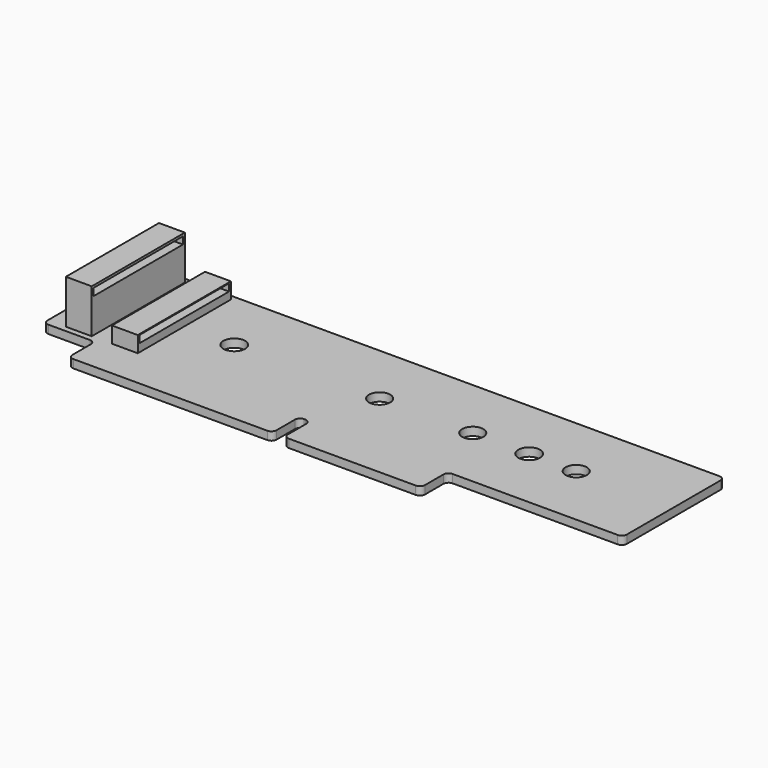
from build123d import *

# Parameters (mm, degrees)
F4_W         = 39.45
F4_H         = 6.43
F4_W_2       = 26.5
F4_R         = 2.105
F4_R_2       = 2.05
F5_DEPTH     = 1.6
F7_DEPTH     = 3.1
F6_W         = 5
F6_H         = 22.5
F8_DEPTH     = 8.5
F9_R         = 1
F10_W        = 21.6
F10_H        = 1.4
F11_DEPTH    = 3.1
F12_T1_DEPTH = 21.6
F13_W        = 21.6
F13_H        = 1.4
F14_DEPTH    = 3.1
F15_T1_DEPTH = 21.6


# Not quite as in the source:
# - a fillet or chamfer that OpenCascade refuses, or shapes differently, is made with other operations: its cross-section is extruded or revolved along the edge and cut away or added
# - a feature names something its author has since deleted; it is built from what else it names


with BuildPart() as f5:
    # F4 (on Top) → F5 (new body)
    with BuildSketch(Plane.XY):
        with Locations((2.695, -15.585)):
            Rectangle(F4_W, F4_H)
        with Locations((37.87, -15.585)):
            Rectangle(F4_W_2, F4_H)
        Polygon((85, 12.23), (-27, 12.23), (-27, -12.37), (-17.03, -12.37), (22.42, -12.37), (24.62, -12.37), (51.12, -12.37), (85, -12.37), align=None)
        Circle(F4_R, mode=Mode.SUBTRACT)
        with Locations((28.1, 0)):
            Circle(F4_R_2, mode=Mode.SUBTRACT)
        with Locations((46.1, 0)):
            Circle(F4_R_2, mode=Mode.SUBTRACT)
        with Locations((57, 0)):
            Circle(F4_R, mode=Mode.SUBTRACT)
        with Locations((66.1, 0)):
            Circle(F4_R_2, mode=Mode.SUBTRACT)
    extrude(amount=F5_DEPTH)

    # F6 (on face) → F7 (join)
    with BuildSketch(Plane.XY.offset(1.6)):
        Polygon((-9.65, 11.25), (-14.65, 11.25), (-14.65, -11.25), (-9.65, -11.25), (-9.65, 0), align=None)
    extrude(amount=F7_DEPTH)

    # F6 (on face) → F8 (join)
    with BuildSketch(Plane.XY.offset(1.6)):
        with Locations((-21.05, 0)):
            Rectangle(F6_W, F6_H)
    extrude(amount=F8_DEPTH)

    # F9
    f9_edges = [f5.edges().sort_by_distance(p)[0] for p in [
        (-27, -12.37, 0.8),
        (-17.03, -12.37, 0.8),
        (-17.03, -18.8, 0.8),
        (24.62, -12.37, 0.8),
        (24.62, -18.8, 0.8),
        (22.42, -18.8, 0.8),
        (51.12, -18.8, 0.8),
        (22.42, -12.37, 0.8),
        (51.12, -12.37, 0.8),
        (85, 12.23, 0.8),
        (-27, 12.23, 0.8),
        (85, -12.37, 0.8),
    ]]
    fillet(f9_edges, radius=F9_R)

    # F10 (on face) → F11 (cut)
    with BuildSketch(Plane.YZ.offset(-9.65)):
        with Locations((0, 3.84)):
            Rectangle(F10_W, F10_H)
    extrude(amount=-F11_DEPTH, mode=Mode.SUBTRACT)

    # F12: fillet of radius 2 on 1 edges, made by hand

    # F12_s2 → F12_t1 (join)
    with BuildSketch(Plane.XZ.offset(-10.8)):
        with BuildLine():
            ThreePointArc((-10.8421215972, 4.54), (-12.0253375538, 4.1524515497), (-12.75, 3.14))
            Line((-12.75, 3.14), (-12.75, 4.54))
            Line((-12.75, 4.54), (-10.8421215972, 4.54))
        make_face()
    extrude(amount=F12_T1_DEPTH)

    # F13 (on face) → F14 (cut)
    with BuildSketch(Plane.YZ.offset(-18.55)):
        with Locations((0, 8.95)):
            Rectangle(F13_W, F13_H)
    extrude(amount=-F14_DEPTH, mode=Mode.SUBTRACT)

    # F15: fillet of radius 2 on 1 edges, made by hand

    # F15_s2 → F15_t1 (join)
    with BuildSketch(Plane.XZ.offset(-10.8)):
        with BuildLine():
            ThreePointArc((-19.7421215972, 9.65), (-20.9253375538, 9.2624515497), (-21.65, 8.25))
            Line((-21.65, 8.25), (-21.65, 9.65))
            Line((-21.65, 9.65), (-19.7421215972, 9.65))
        make_face()
    extrude(amount=F15_T1_DEPTH)


solid = f5.part
